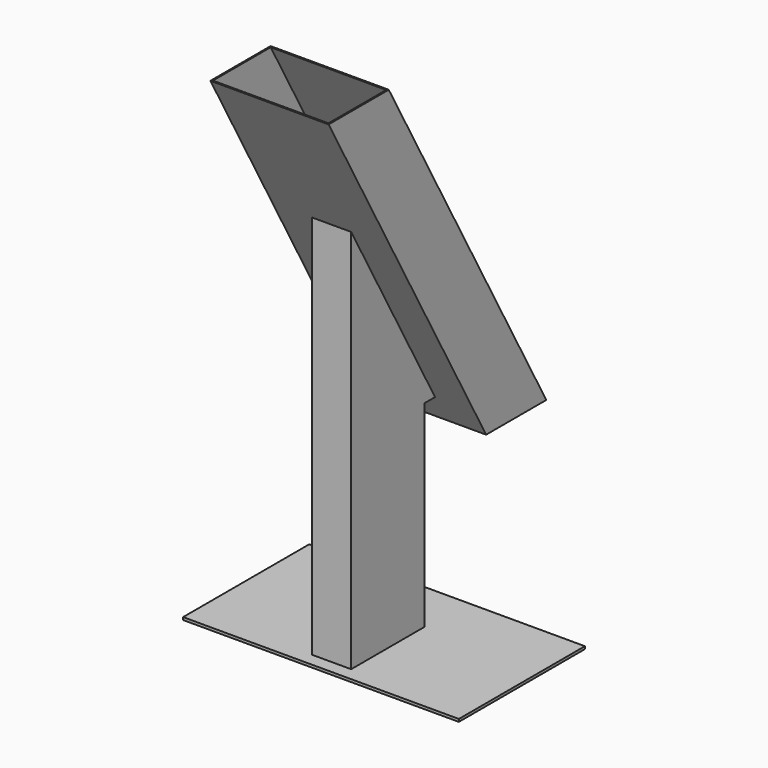
from build123d import *

# Parameters (mm, degrees)
F1_DEPTH   = 228.6
F2_T       = -2.54
F4_W       = 223.52
F4_H       = 121.926114556
F5_DEPTH   = 134.112
F7_W       = 76.2
F7_H       = 177.8
F9_W       = 76.2
F9_H       = 177.8
F10_DEPTH  = 381
F8_FACE1_W = 76.2
F8_FACE1_H = 103.6678810409
F13_T      = -2.54
F11_W      = 533.4
F11_H      = 304.8
F11_W_2    = 76.2
F11_H_2    = 177.8
F14_DEPTH  = 5.08


# Not quite as in the source:
# - a shell that OpenCascade refuses in one call is made with other operations: the cavity is built on its own and cut out
# - a feature names something its author has since deleted; it is built from what else it names


with BuildPart() as f1:
    # F0 (on Right) → F1 (new body)
    with BuildSketch(Plane.YZ):
        Polygon((-381, 683.26), (0, 0), (145.4103401064, 0), (-235.5896598936, 683.26), align=None)
    extrude(amount=F1_DEPTH)

    # F2
    f2_openings = [f1.faces().sort_by_distance(p)[0] for p in [
        (114.3, -308.29483, 683.26),
    ]]
    offset(amount=F2_T, openings=f2_openings)

    # F4 (on face) → F5 (cut)
    with BuildSketch(Plane(origin=(0, 34.4790739886, -61.8450267372), x_dir=(1, 0, 0), z_dir=(0, -0.4869452699, 0.873432484))):
        with Locations((114.3, 63.503057278)):
            Rectangle(F4_W, F4_H)
    extrude(amount=F5_DEPTH, mode=Mode.SUBTRACT)

    # F7 (on offset) → F8 (join, up to the next surface of F1)
    with BuildSketch(Plane.XZ.offset(231.14)):
        with Locations((114.3, 139.7)):
            Rectangle(F7_W, F7_H)
    extrude(until=Until.NEXT, dir=(0, 1, 0))

    # F9 (on face) → F10 (join)
    with BuildSketch(Plane(origin=(0, 0, 50.8), x_dir=(1, 0, 0), z_dir=(0, 0, -1))):
        with Locations((114.3, 142.24)):
            Rectangle(F9_W, F9_H)
    extrude(amount=F10_DEPTH)

    # F8_face1 (on face) → F12 (join, up to the next surface of F1)
    with BuildSketch(Plane(origin=(114.3, -179.3060594796, 228.6), x_dir=(1, 0, 0), z_dir=(0, 0, 1))):
        Rectangle(F8_FACE1_W, F8_FACE1_H)
    extrude(until=Until.NEXT)

    # F13: a shell. OpenCascade refuses it in one call, so the cavity is built on its own and cut out:
    # the body offset inwards by the wall thickness, plus a prism from it out through each open face.
    f13_core = offset(f1.part, amount=F13_T, kind=Kind.INTERSECTION, mode=Mode.PRIVATE)
    f13_exits = [f13_core.faces().sort_by_distance(p)[0] for p in [
        (114.3, -55.88, -137.16),
    ]]
    add(f13_core, mode=Mode.SUBTRACT)
    extrude(f13_exits, amount=-F13_T, mode=Mode.SUBTRACT)

    # F11 (on face) → F14 (join)
    with BuildSketch(Plane(origin=(0, 0, -330.2), x_dir=(1, 0, 0), z_dir=(0, 0, -1))):
        with Locations((114.3, 104.14)):
            Rectangle(F11_W, F11_H)
        with Locations((114.3, 142.24)):
            Rectangle(F11_W_2, F11_H_2, mode=Mode.SUBTRACT)
        with Locations((114.3, 142.24)):
            Rectangle(F11_W_2, F11_H_2)
    extrude(amount=F14_DEPTH)


solid = f1.part
